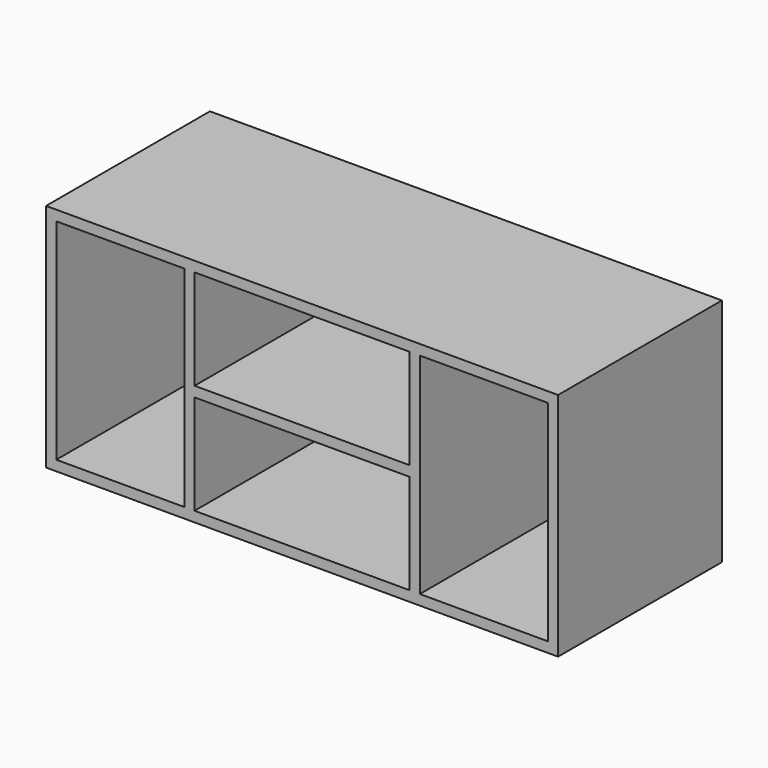
from build123d import *

# Parameters (mm, degrees)
F0_W     = 1000
F0_H     = 450
F0_W_2   = 250
F0_H_2   = 410
F0_W_3   = 420
F1_DEPTH = 200
F2_W     = 400
F2_H     = 20
F3_DEPTH = 420


# Not quite as in the source:
# - a feature names something its author has since deleted; it is built from what else it names


with BuildPart() as f1:
    # F0 (on Front) → F1 (new body, symmetric)
    with BuildSketch(Plane.XZ):
        Rectangle(F0_W, F0_H)
        with Locations((-355, 0)):
            Rectangle(F0_W_2, F0_H_2, mode=Mode.SUBTRACT)
        Rectangle(F0_W_3, F0_H_2, mode=Mode.SUBTRACT)
        with Locations((355, 0)):
            Rectangle(F0_W_2, F0_H_2, mode=Mode.SUBTRACT)
    extrude(amount=F1_DEPTH, both=True)

    # F2 (on face) → F3 (join, through all)
    with BuildSketch(Plane(origin=(210, 0, 0), x_dir=(0, -1, 0), z_dir=(-1, 0, 0))):
        Rectangle(F2_W, F2_H)
    extrude(amount=F3_DEPTH)


solid = f1.part
